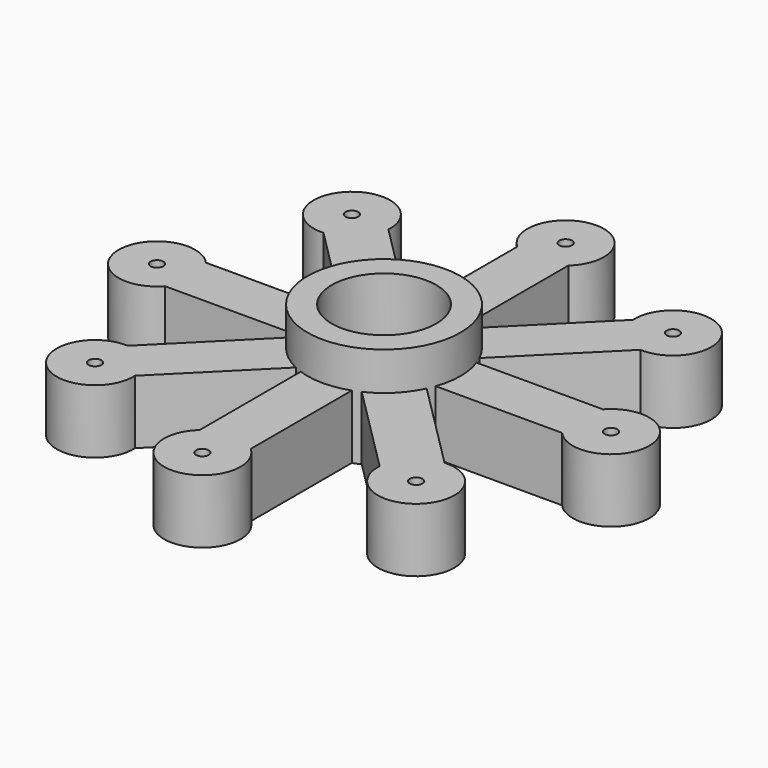
from build123d import *

# Parameters (mm, degrees)
F1_R            = 6
F2_DEPTH        = 8
F0_R            = 0.5
F3_DEPTH        = 5
F3_COPIES_COUNT = 8
F4_R            = 4.1
F5_DEPTH        = 8.001


# Not quite as in the source:
# - a pattern or mirror of a feature is missing from the dataset's text; its kind, count and spacing are read off the source's solid


with BuildPart() as f2:
    # F1 (on Top) → F2 (new body)
    with BuildSketch(Plane.XY):
        Circle(F1_R)
    extrude(amount=F2_DEPTH)

    # F0 (on Top) → F3 (join)
    with BuildSketch(Plane.XY):
        with BuildLine():
            Line((0, 2), (-15.5639320225, 2))
            ThreePointArc((-15.5639320225, 2), (-20.8, 0), (-15.5639320225, -2))
            Line((-15.5639320225, -2), (0, -2))
            Line((0, -2), (0, 2))
        make_face()
        with Locations((-17.8, 0)):
            Circle(F0_R, mode=Mode.SUBTRACT)
    f3 = extrude(amount=F3_DEPTH)

    # F3_copies: F3 ×8 about axis
    f3_copies_axis = Axis((0, 0, 0), (0, 0, 1))
    for i in range(1, F3_COPIES_COUNT):
        add(f3.rotate(f3_copies_axis, i * 360 / F3_COPIES_COUNT))

    # F4 (on Top) → F5 (cut, through all)
    with BuildSketch(Plane.XY):
        Circle(F4_R)
    extrude(amount=F5_DEPTH, mode=Mode.SUBTRACT)


solid = f2.part
